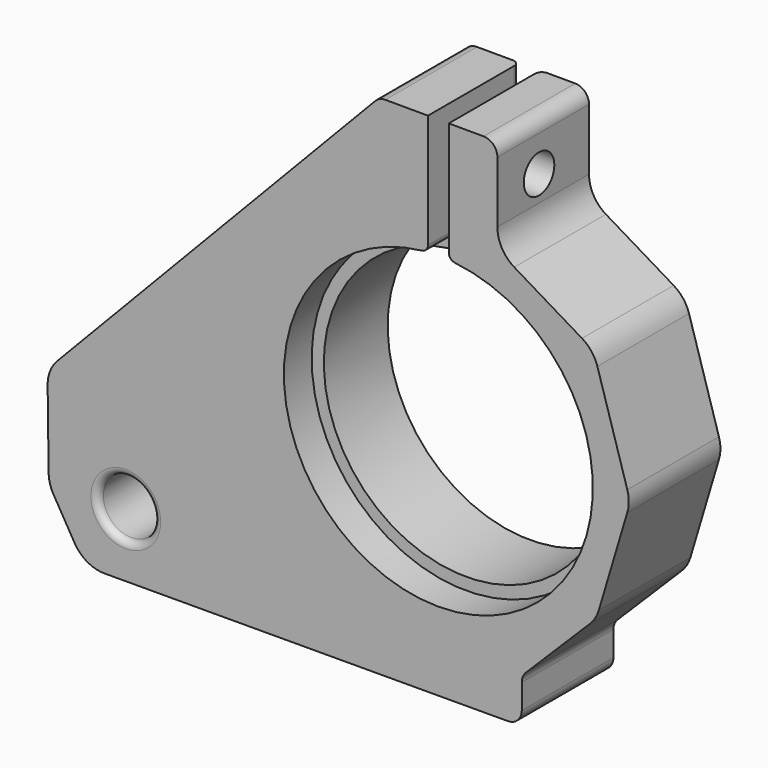
from build123d import *

# Parameters (mm, degrees)
F15_DEPTH = 16.5
F16_R     = 20.5
F17_DEPTH = 16.5
F18_R     = 4.0274870607
F19_DEPTH = 16.5
F20_W     = 3
F20_H     = 20
F21_DEPTH = 16.5
F22_R     = 2.75
F23_DEPTH = 40
F26_DEPTH = 31.3
F27_R     = 22.25
F28_DEPTH = 5
F29_R     = 1
F30_R     = 5
F31_R     = 5
F32_R     = 5
F33_R     = 5
F34_R     = 5
F35_R     = 2
F36_R     = 2


# Not quite as in the source:
# - a feature of the source that left no trace in its solid (it failed there, or was rolled back) is left out


with BuildPart() as f15:
    # F14 (on offset) → F15 (new body)
    with BuildSketch(Plane.XZ.offset(20)):
        Polygon((8.5, 39.5), (-8.5, 39.5365608335), (-56.3052967191, -10.4271536693), (-56.1165139079, -24.8827897012), (-50.9412027895, -33.6846895516), (12.0133129929, -33.5), (12.0133129929, -27.1025877446), (22.7434113622, -16.4029654115), (27.6456046849, 0), (22.3432332277, 17.5122059882), (8.5, 25.806048885), align=None)
    extrude(amount=F15_DEPTH)

    # F16 (on face) → F17 (cut)
    with BuildSketch(Plane.XZ.offset(36.5)):
        Circle(F16_R)
    extrude(amount=-F17_DEPTH, mode=Mode.SUBTRACT)

    # F18 (on face) → F19 (cut)
    with BuildSketch(Plane.XZ.offset(36.5)):
        with Locations((-45.0200997293, -24.5124399662)):
            Circle(F18_R)
    extrude(amount=-F19_DEPTH, mode=Mode.SUBTRACT)

    # F20 (on face) → F21 (cut)
    with BuildSketch(Plane.XZ.offset(36.5)):
        with Locations((0, 30.4450483003)):
            Rectangle(F20_W, F20_H)
    extrude(amount=-F21_DEPTH, mode=Mode.SUBTRACT)

    # F22 (on face) → F23 (cut)
    with BuildSketch(Plane.YZ.offset(8.5)):
        with Locations((-29, 32.35)):
            Circle(F22_R)
    extrude(amount=-F23_DEPTH, mode=Mode.SUBTRACT)

    # F25 (on offset) → F26 (cut)
    with BuildSketch(Plane.YZ.offset(-36.7)):
        Polygon((-32.875, 34.5872322931), (-32.875, 30.1127677069), (-29, 27.8755354138), (-25.125, 30.1127677069), (-25.125, 34.5872322931), (-29, 36.8244645862), align=None)
    extrude(amount=F26_DEPTH, mode=Mode.SUBTRACT)

    # F27 (on face) → F28 (cut)
    with BuildSketch(Plane.XZ.offset(36.5)):
        Circle(F27_R)
    extrude(amount=-F28_DEPTH, mode=Mode.SUBTRACT)

    # F29
    f29_edges = [f15.edges().sort_by_distance(p)[0] for p in [
        (-49.047587, -36.5, -24.51244),
        (-1.5, -20, 29.983277),
        (1.5, -20, 29.980051),
        (-1.5, -34, 22.199381),
        (-1.5, -31.5, 21.322214),
        (-1.5, -25.75, 20.445048),
        (1.5, -25.75, 20.445048),
        (1.5, -31.5, 21.322214),
        (1.5, -34, 22.199381),
    ]]
    fillet(f29_edges, radius=F29_R)

    # F30
    f30_edges = [f15.edges().sort_by_distance(p)[0] for p in [
        (27.645605, -28.25, 0),
    ]]
    fillet(f30_edges, radius=F30_R)

    # F31
    f31_edges = [f15.edges().sort_by_distance(p)[0] for p in [
        (22.343233, -28.25, 17.512206),
    ]]
    fillet(f31_edges, radius=F31_R)

    # F32
    f32_edges = [f15.edges().sort_by_distance(p)[0] for p in [
        (22.743411, -28.25, -16.402965),
    ]]
    fillet(f32_edges, radius=F32_R)

    # F33
    f33_edges = [f15.edges().sort_by_distance(p)[0] for p in [
        (8.5, -28.25, 25.806049),
    ]]
    fillet(f33_edges, radius=F33_R)

    # F34
    f34_edges = [f15.edges().sort_by_distance(p)[0] for p in [
        (-50.941203, -28.25, -33.68469),
        (-56.116514, -28.25, -24.88279),
        (-56.305297, -28.25, -10.427154),
    ]]
    fillet(f34_edges, radius=F34_R)

    # F35
    f35_edges = [f15.edges().sort_by_distance(p)[0] for p in [
        (12.013313, -28.25, -33.5),
        (12.013313, -28.25, -27.102588),
    ]]
    fillet(f35_edges, radius=F35_R)

    # F36
    f36_edges = [f15.edges().sort_by_distance(p)[0] for p in [
        (-8.5, -28.25, 39.536561),
        (8.5, -28.25, 39.5),
    ]]
    fillet(f36_edges, radius=F36_R)


solid = f15.part
